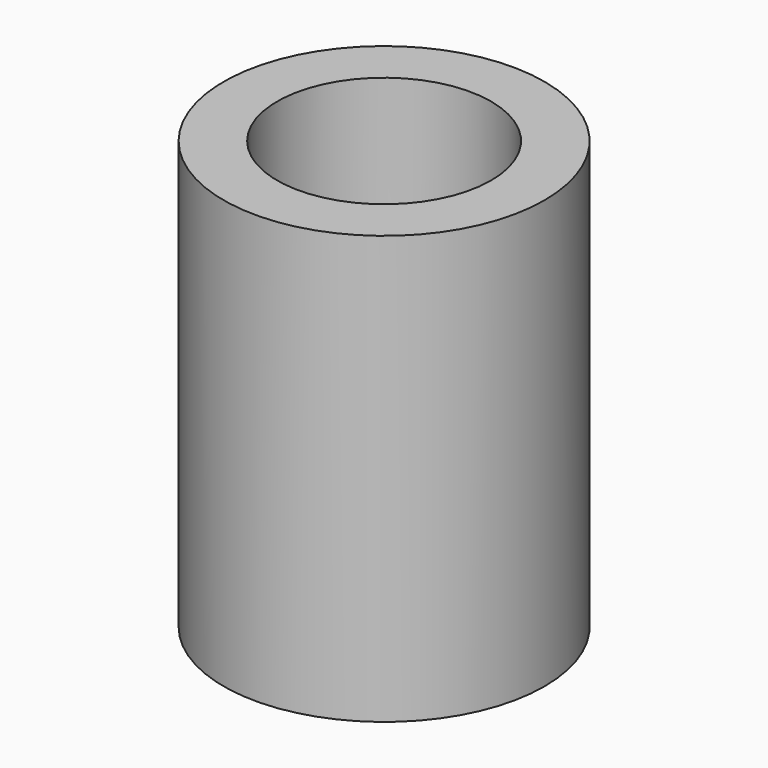
from build123d import *

# Parameters (mm, degrees)
F0_R     = 15
F0_R_2   = 10
F1_DEPTH = 40


# Not quite as in the source:
# - the program builds the solid bodies; features that only make, move or delete a surface that nothing else refers to are left out


with BuildPart() as f1:
    # F0 (on Top) → F1 (new body)
    with BuildSketch(Plane.XY):
        Circle(F0_R)
        Circle(F0_R_2, mode=Mode.SUBTRACT)
    extrude(amount=F1_DEPTH)


solid = f1.part
